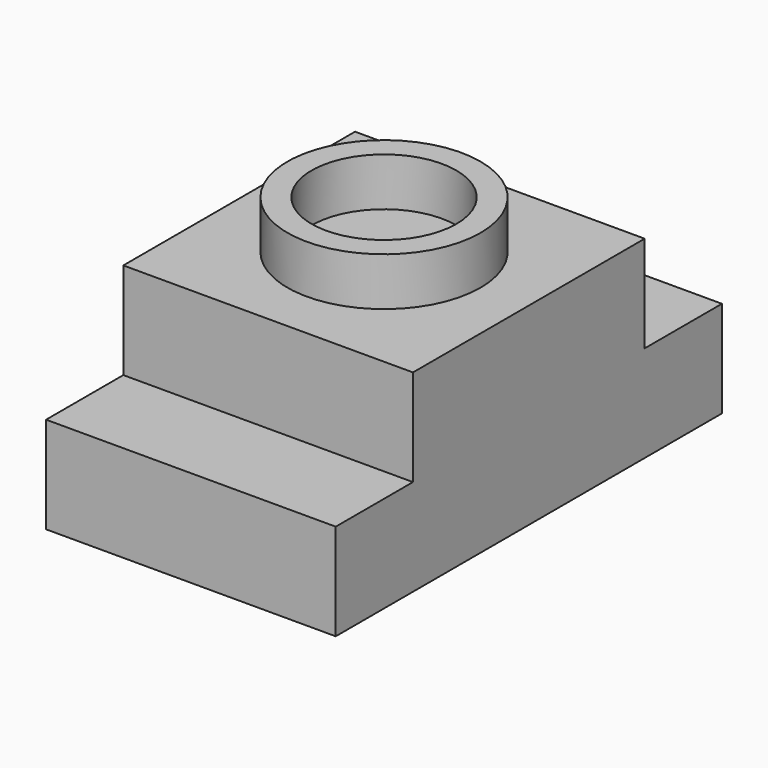
from build123d import *

# Parameters (mm, degrees)
F1_DEPTH = 38.1
F2_R     = 12.7
F2_R_2   = 9.525
F3_DEPTH = 6.35


# Not quite as in the source:
# - a feature names something its author has since deleted; it is built from what else it names


with BuildPart() as f1:
    # F0 (on Right) → F1 (new body)
    with BuildSketch(Plane.YZ):
        Polygon((-31.75, 0), (0, 0), (31.75, 0), (31.75, 12.7), (19.05, 12.7), (19.05, 25.4), (-19.05, 25.4), (-19.05, 12.7), (-31.75, 12.7), align=None)
    extrude(amount=F1_DEPTH)

    # F2 (on face) → F3 (join)
    with BuildSketch(Plane.XY.offset(25.4)):
        with Locations((19.05, 0)):
            Circle(F2_R)
        with Locations((19.05, 0)):
            Circle(F2_R_2, mode=Mode.SUBTRACT)
    extrude(amount=F3_DEPTH)


solid = f1.part
